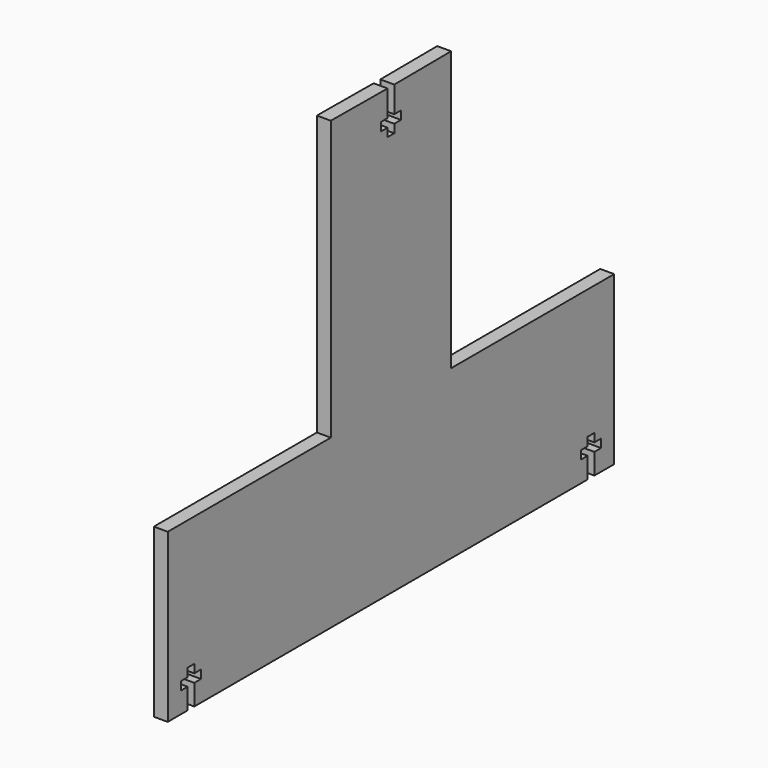
from build123d import *

# Parameters (mm, degrees)
F1_DEPTH = 2.5


# Not quite as in the source:
# - a feature names something its author has since deleted; it is built from what else it names


with BuildPart() as f1:
    # F0 (on Right) → F1 (new body)
    with BuildSketch(Plane.YZ):
        Polygon((45.5622866154, 0), (50, -0.0115907192), (50, 29.9884092808), (13.482012786, 29.9884092808), (13.482012786, 79.9884092808), (0.7398080197, 79.910288877), (0.7398080197, 75.2277448773), (2.2398080197, 75.2277448773), (2.2398080197, 73.7277448773), (0.7398080197, 73.7277448773), (0.7398080197, 72.2277448773), (-0.7601919803, 72.2277448773), (-0.7601919803, 73.7277448773), (-2.2601919803, 73.7277448773), (-2.2601919803, 75.2277448773), (-0.7601919803, 75.2277448773), (-0.7601919803, 79.9100687942), (-13.482012786, 79.9884092808), (-13.482012786, 29.9884092808), (-50, 29.9884092808), (-50, -0.0115907192), (-45.5622866154, 0), (-45.5622866154, 3.739590158), (-47.0622866154, 3.739590158), (-47.0622866154, 5.239590158), (-45.5622866154, 5.239590158), (-45.5622866154, 6.739590158), (-44.0622866154, 6.739590158), (-44.0622866154, 5.239590158), (-42.5622866154, 5.239590158), (-42.5622866154, 3.739590158), (-44.0622866154, 3.739590158), (-44.0622866154, 0), (0, 0), (44.0622866154, 0), (44.0622866154, 3.739590158), (42.5622866154, 3.739590158), (42.5622866154, 5.239590158), (44.0622866154, 5.239590158), (44.0622866154, 6.739590158), (45.5622866154, 6.739590158), (45.5622866154, 5.239590158), (47.0622866154, 5.239590158), (47.0622866154, 3.739590158), (45.5622866154, 3.739590158), align=None)
    extrude(amount=F1_DEPTH)


solid = f1.part
